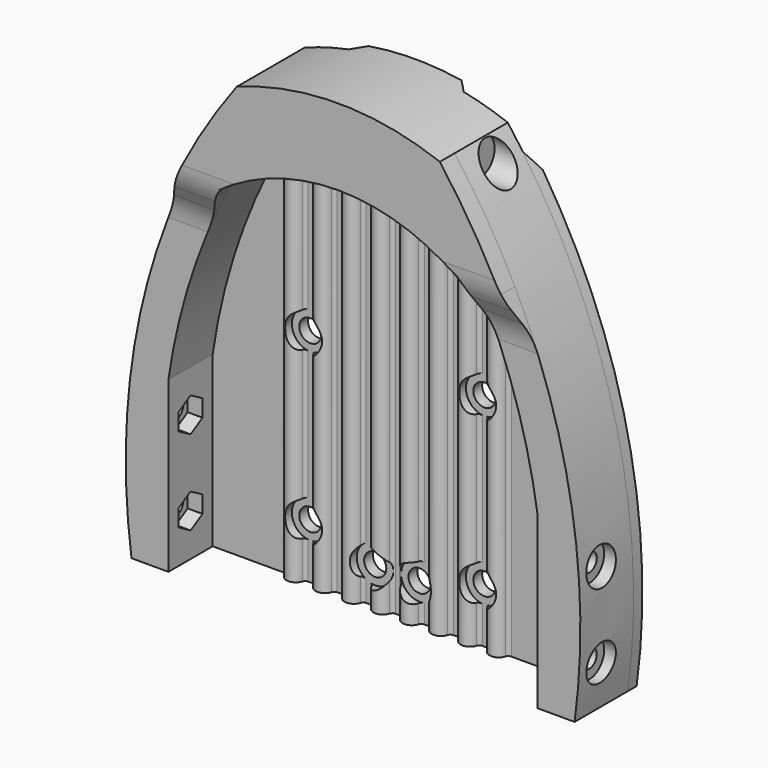
from build123d import *

# Parameters (mm, degrees)
F2_DEPTH       = 3
F4_DEPTH       = 15
F7_R           = 1
F11_R          = 5
F12_DEPTH      = 5
F12_DEPTH_BACK = 25
F13_R          = 5
F14_DEPTH      = 5
F14_DEPTH_BACK = 25
F15_R          = 3
F16_DEPTH      = 25
F17_R          = 5
F18_DEPTH      = 25
F20_DEPTH      = 3
F21_SIZE       = 2.99999
F23_DEPTH      = 5
F25_DEPTH      = 61.5543717068
F25_DEPTH_BACK = 61.5543717068
F26_T4_DEPTH   = 11.3646029343
F26_S5_R       = 15
F26_T6_DEPTH   = 8
F26_T10_DEPTH  = 11.3646029343
F26_S11_R      = 15
F26_T12_DEPTH  = 8
F27_R          = 2.5
F28_DEPTH      = 25
F28_DEPTH_BACK = 111.5543717068
F30_DEPTH      = 4
F32_DEPTH      = 4
F34_R          = 5
F35_DEPTH      = 25
F37_R          = 5
F38_DEPTH      = 25


# Not quite as in the source:
# - a fillet or chamfer that OpenCascade refuses, or shapes differently, is made with other operations: its cross-section is extruded or revolved along the edge and cut away or added
# - a fillet or chamfer is up to 0.001 mm smaller than in the source, because OpenCascade refuses the exact size
# - a feature names something its author has since deleted; it is built from what else it names


with BuildPart() as f2:
    # F1 (on Front) → F2 (new body)
    with BuildSketch(Plane.XZ):
        with BuildLine():
            ThreePointArc((0, 130), (-13.9754248594, 128.7398367266), (-27.5, 125))
            ThreePointArc((-27.5, 125), (-56.0831977608, 65.7066314178), (-60, 0))
            Line((-60, 0), (0, 0))
            Line((0, 0), (60, 0))
            ThreePointArc((60, 0), (56.0831977608, 65.7066314178), (27.5, 125))
            ThreePointArc((27.5, 125), (13.9754248594, 128.7398367266), (0, 130))
        make_face()
    extrude(amount=F2_DEPTH)

    # F3 (on face) → F4 (join)
    with BuildSketch(Plane.XZ.offset(3)):
        with BuildLine():
            ThreePointArc((60, 0), (56.0831977608, 65.7066314178), (27.5, 125))
            ThreePointArc((27.5, 125), (0, 130), (-27.5, 125))
            ThreePointArc((-27.5, 125), (-56.0831977608, 65.7066314178), (-60, 0))
            Line((-60, 0), (-50, 0))
            ThreePointArc((-50, 0), (-51.6504278949, 22.9288766178), (-50, 45.8577532355))
            ThreePointArc((-50, 45.8577532355), (-42.4331694009, 76.4672184834), (-29.0139046296, 105))
            ThreePointArc((-29.0139046296, 105), (0, 114.2790798465), (29.0139046296, 105))
            ThreePointArc((29.0139046296, 105), (42.4331694009, 76.4672184834), (50, 45.8577532355))
            ThreePointArc((50, 45.8577532355), (51.6504278949, 22.9288766178), (50, 0))
            Line((50, 0), (60, 0))
        make_face()
        with BuildLine():
            Line((50, 45.8577532355), (50, 0))
            ThreePointArc((50, 0), (51.6504278949, 22.9288766178), (50, 45.8577532355))
        make_face()
        with BuildLine():
            ThreePointArc((-50, 45.8577532355), (-51.6504278949, 22.9288766178), (-50, 0))
            Line((-50, 0), (-50, 45.8577532355))
        make_face()
    extrude(amount=F4_DEPTH)

    # F5 (on face) → F6 (join, up to the next surface of F2)
    with BuildSketch(Plane(origin=(0, 0, 0), x_dir=(1, 0, 0), z_dir=(0, 0, -1))):
        with BuildLine():
            Line((-30, 3), (-25, 3))
            ThreePointArc((-25, 3), (-27.5, 5.5), (-30, 3))
        make_face()
        with BuildLine():
            Line((-22.1428571429, 3), (-17.1428571429, 3))
            ThreePointArc((-17.1428571429, 3), (-19.6428571429, 5.5), (-22.1428571429, 3))
        make_face()
        with BuildLine():
            Line((-14.2857142857, 3), (-9.2857142857, 3))
            ThreePointArc((-9.2857142857, 3), (-11.7857142857, 5.5), (-14.2857142857, 3))
        make_face()
        with BuildLine():
            Line((-6.4285714286, 3), (-1.4285714286, 3))
            ThreePointArc((-1.4285714286, 3), (-3.9285714286, 5.5), (-6.4285714286, 3))
        make_face()
        with BuildLine():
            Line((1.4285714286, 3), (6.4285714286, 3))
            ThreePointArc((6.4285714286, 3), (3.9285714286, 5.5), (1.4285714286, 3))
        make_face()
        with BuildLine():
            Line((9.2857142857, 3), (14.2857142857, 3))
            ThreePointArc((14.2857142857, 3), (11.7857142857, 5.5), (9.2857142857, 3))
        make_face()
        with BuildLine():
            Line((17.1428571429, 3), (22.1428571429, 3))
            ThreePointArc((22.1428571429, 3), (19.6428571429, 5.5), (17.1428571429, 3))
        make_face()
        with BuildLine():
            Line((25, 3), (30, 3))
            ThreePointArc((30, 3), (27.5, 5.5), (25, 3))
        make_face()
    extrude(until=Until.NEXT, dir=(0, 0, 1))

    # F7
    f7_edges = [f2.edges().sort_by_distance(p)[0] for p in [
        (-30, -3, 51.662692),
        (-25, -3, 53.790175),
        (-17.142857, -3, 55.624229),
        (-9.285714, -3, 56.704635),
        (-1.428571, -3, 57.129334),
        (6.428571, -3, 56.932046),
        (14.285714, -3, 56.097411),
        (22.142857, -3, 54.554345),
        (30, -3, 51.662692),
        (-22.142857, -3, 54.554345),
        (-14.285714, -3, 56.097411),
        (-6.428571, -3, 56.932046),
        (1.428571, -3, 57.129334),
        (9.285714, -3, 56.704635),
        (17.142857, -3, 55.624229),
        (25, -3, 53.790175),
    ]]
    fillet(f7_edges, radius=F7_R)

    # F11 (on offset) → F12 (cut, two sides)
    with BuildSketch(Plane.YZ.offset(31.337)) as f12_sk:
        with Locations((-8, 119.67874604)):
            Circle(F11_R)
    extrude(amount=-F12_DEPTH, mode=Mode.SUBTRACT)
    extrude(f12_sk.sketch, amount=F12_DEPTH_BACK, mode=Mode.SUBTRACT)

    # F13 (on offset) → F14 (cut, two sides)
    with BuildSketch(Plane.YZ.offset(-31.337)) as f14_sk:
        with Locations((-8, 119.67874604)):
            Circle(F13_R)
    extrude(amount=F14_DEPTH, mode=Mode.SUBTRACT)
    extrude(f14_sk.sketch, amount=-F14_DEPTH_BACK, mode=Mode.SUBTRACT)

    # F15 (on face) → F16 (cut)
    with BuildSketch(Plane.XZ.offset(3)):
        with Locations((-23.5714285714, 15)):
            Circle(F15_R)
        with Locations((-23.5714285714, 60)):
            Circle(F15_R)
        with Locations((23.5714285714, 15)):
            Circle(F15_R)
        with Locations((23.5714285714, 60)):
            Circle(F15_R)
        with Locations((6, 10)):
            Circle(F15_R)
        with Locations((-6, 10)):
            Circle(F15_R)
    extrude(amount=-F16_DEPTH, mode=Mode.SUBTRACT)

    # F17 (on face) → F18 (cut)
    with BuildSketch(Plane.XZ.offset(3)):
        with Locations((23.5714285714, 60)):
            Circle(F17_R)
        with Locations((-23.5714285714, 60)):
            Circle(F17_R)
        with Locations((-23.5714285714, 15)):
            Circle(F17_R)
        with Locations((23.5714285714, 15)):
            Circle(F17_R)
        with Locations((6, 10)):
            Circle(F17_R)
        with Locations((-6, 10)):
            Circle(F17_R)
    extrude(amount=F18_DEPTH, mode=Mode.SUBTRACT)

    # F19 (on face) → F20 (join)
    with BuildSketch(Plane(origin=(0, 0, 0), x_dir=(-1, 0, 0), z_dir=(0, 1, 0))):
        with BuildLine():
            Line((-15.5714285714, 23.0840109289), (15.5714285714, 23.0840109289))
            Line((15.5714285714, 23.0840109289), (15.5714285714, 128.4324701596))
            ThreePointArc((15.5714285714, 128.4324701596), (0, 130), (-15.5714285714, 128.4324701596))
            Line((-15.5714285714, 128.4324701596), (-15.5714285714, 23.0840109289))
        make_face()
        with BuildLine():
            Line((31.5714285714, 0), (60, 0))
            ThreePointArc((60, 0), (56.9259044213, 62.3233608827), (31.5714285714, 119.3391650928))
            Line((31.5714285714, 119.3391650928), (31.5714285714, 0))
        make_face()
        with BuildLine():
            ThreePointArc((-31.5714285714, 119.3391650928), (-56.9259044213, 62.3233608827), (-60, 0))
            Line((-60, 0), (-31.5714285714, 0))
            Line((-31.5714285714, 0), (-31.5714285714, 119.3391650928))
        make_face()
    extrude(amount=F20_DEPTH)

    # F21 (size 3 in the source; OpenCascade refuses exactly that, so slightly less here)
    f21_edges = [f2.edges().sort_by_distance(p)[0] for p in [
        (-15.571429, 3, 75.758241),
        (15.571429, 3, 75.758241),
        (31.571429, 3, 59.669583),
        (-31.571429, 3, 59.669583),
        (0, 3, 23.084011),
    ]]
    chamfer(f21_edges, length=F21_SIZE)

    # F22 (on face) → F23 (join)
    with BuildSketch(Plane.XZ.offset(18)):
        with BuildLine():
            ThreePointArc((43.8257492004, 98.5140803416), (36.2700770628, 112.131315833), (27.5, 125))
            ThreePointArc((27.5, 125), (0, 130), (-27.5, 125))
            ThreePointArc((-27.5, 125), (-36.2700770628, 112.131315833), (-43.8257492004, 98.5140803416))
            ThreePointArc((-43.8257492004, 98.5140803416), (-47.2891381531, 91.0931709237), (-50.3911287357, 83.5140803416))
            Line((-50.3911287357, 83.5140803416), (-39.7441288148, 83.5140803416))
            ThreePointArc((-39.7441288148, 83.5140803416), (-36.4085138648, 91.1055235986), (-32.6843193474, 98.5140803416))
            ThreePointArc((-32.6843193474, 98.5140803416), (0, 109.2790798465), (32.6843193474, 98.5140803416))
            ThreePointArc((32.6843193474, 98.5140803416), (36.4085138648, 91.1055235986), (39.7441288148, 83.5140803416))
            Line((39.7441288148, 83.5140803416), (50.3911287357, 83.5140803416))
            ThreePointArc((50.3911287357, 83.5140803416), (47.2891381531, 91.0931709237), (43.8257492004, 98.5140803416))
        make_face()
    extrude(amount=F23_DEPTH)

    # F24 (on Right) → F25 (cut, two sides)
    with BuildSketch(Plane.YZ) as f25_sk:
        with BuildLine():
            ThreePointArc((-18, 84.5140803416), (-18.4177080594, 88.0292989349), (-19.6475682345, 91.34873951))
            Line((-19.6475682345, 91.34873951), (-21.3524317655, 94.6794211731))
            ThreePointArc((-21.3524317655, 94.6794211731), (-22.5822919406, 97.9988617482), (-23, 101.5140803416))
            Line((-23, 101.5140803416), (-23, 105.4066538624))
            Line((-23, 105.4066538624), (-29.6550593126, 105.4066538624))
            Line((-29.6550593126, 105.4066538624), (-29.6550593126, 83.5140803416))
            Line((-29.6550593126, 83.5140803416), (-18, 83.5140803416))
            Line((-18, 83.5140803416), (-18, 84.5140803416))
        make_face()
    extrude(amount=-F25_DEPTH, mode=Mode.SUBTRACT)
    extrude(f25_sk.sketch, amount=F25_DEPTH_BACK, mode=Mode.SUBTRACT)

    # F26: fillet of radius 10 on 2 edges, made by hand


with BuildPart() as f26_tool2:
    # F26_s3 → F26_t4 (new body)
    with BuildSketch(Plane.XZ.offset(18)):
        with BuildLine():
            ThreePointArc((-30.5014733129, 100.0465369066), (-32.4105610498, 98.390449678), (-33.8434921036, 96.3086356875))
            ThreePointArc((-33.8434921036, 96.3086356875), (-33.2681960845, 97.4136130098), (-32.6843193474, 98.5140803416))
            ThreePointArc((-32.6843193474, 98.5140803416), (-31.6021867014, 99.2935419192), (-30.5014733129, 100.0465369066))
        make_face()
    extrude(amount=F26_T4_DEPTH)

    # F26_s5 → F26_t6 (intersect, symmetric)
    with BuildSketch(Plane.YZ.offset(-32.2)):
        with Locations((-8, 101.5140803416)):
            Circle(F26_S5_R)
    extrude(amount=F26_T6_DEPTH, both=True, mode=Mode.INTERSECT)


with BuildPart() as f2_1:
    add(f2.part)

    # F26_t1: union F26_tool2
    add(f26_tool2.part)


with BuildPart() as f26_tool8:
    # F26_s9 → F26_t10 (new body)
    with BuildSketch(Plane.XZ.offset(18)):
        with BuildLine():
            ThreePointArc((33.8434921036, 96.3086356875), (32.4105610498, 98.390449678), (30.5014733129, 100.0465369066))
            ThreePointArc((30.5014733129, 100.0465369066), (31.6021867014, 99.2935419192), (32.6843193474, 98.5140803416))
            ThreePointArc((32.6843193474, 98.5140803416), (33.2681960845, 97.4136130098), (33.8434921036, 96.3086356875))
        make_face()
    extrude(amount=F26_T10_DEPTH)

    # F26_s11 → F26_t12 (intersect, symmetric)
    with BuildSketch(Plane.YZ.offset(32.2)):
        with Locations((-8, 101.5140803416)):
            Circle(F26_S11_R)
    extrude(amount=F26_T12_DEPTH, both=True, mode=Mode.INTERSECT)


with BuildPart() as f2_2:
    add(f2_1.part)

    # F26_t7: union F26_tool8
    add(f26_tool8.part)

    # F27 (on face) → F28 (cut, two sides)
    with BuildSketch(Plane.YZ.offset(-50)) as f28_sk:
        with Locations((-10.5, 11.4644383089)):
            Circle(F27_R)
        with Locations((-10.5, 34.3933149266)):
            Circle(F27_R)
    extrude(amount=-F28_DEPTH, mode=Mode.SUBTRACT)
    extrude(f28_sk.sketch, amount=F28_DEPTH_BACK, mode=Mode.SUBTRACT)

    # F29 (on face) → F30 (cut)
    with BuildSketch(Plane.YZ.offset(-50)):
        Polygon((-10.5, 16.1121079759), (-14.525, 13.7882731424), (-14.525, 9.1406034754), (-10.5, 6.8167686419), (-6.475, 9.1406034754), (-6.475, 13.7882731424), align=None)
        Polygon((-10.5, 39.0409845936), (-14.525, 36.7171497601), (-14.525, 32.0694800932), (-10.5, 29.7456452597), (-6.475, 32.0694800932), (-6.475, 36.7171497601), align=None)
    extrude(amount=-F30_DEPTH, mode=Mode.SUBTRACT)

    # F31 (on face) → F32 (cut)
    with BuildSketch(Plane(origin=(50, 0, 0), x_dir=(0, -1, 0), z_dir=(-1, 0, 0))):
        Polygon((14.525, 32.0694800932), (14.525, 36.7171497601), (10.5, 39.0409845936), (6.475, 36.7171497601), (6.475, 32.0694800932), (10.5, 29.7456452597), align=None)
        Polygon((14.525, 9.1406034754), (14.525, 13.7882731424), (10.5, 16.1121079759), (6.475, 13.7882731424), (6.475, 9.1406034754), (10.5, 6.8167686419), align=None)
    extrude(amount=-F32_DEPTH, mode=Mode.SUBTRACT)

    # F34 (on offset) → F35 (cut)
    with BuildSketch(Plane.YZ.offset(-58)):
        with Locations((-10.5, 11.4644383089)):
            Circle(F34_R)
        with Locations((-10.5, 34.3933149266)):
            Circle(F34_R)
    extrude(amount=-F35_DEPTH, mode=Mode.SUBTRACT)

    # F37 (on offset) → F38 (cut)
    with BuildSketch(Plane(origin=(58, 0, 0), x_dir=(0, -1, 0), z_dir=(-1, 0, 0))):
        with Locations((10.5, 34.3933149266)):
            Circle(F37_R)
        with Locations((10.5, 11.4644383089)):
            Circle(F37_R)
    extrude(amount=-F38_DEPTH, mode=Mode.SUBTRACT)


solid = f2_2.part
